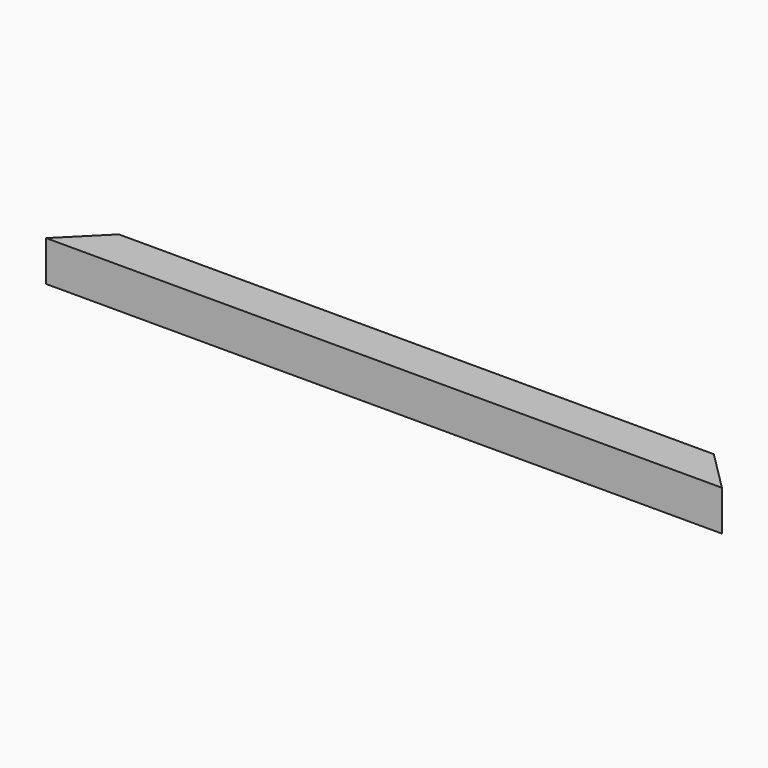
from build123d import *

# Parameters (mm, degrees)
F1_DEPTH = 212.5
F3_DEPTH = 25.4


# Not quite as in the source:
# - a pattern or mirror of a feature is missing from the dataset's text; its kind, count and spacing are read off the source's solid


with BuildPart() as f1:
    # F0 (on Right) → F1 (new body, symmetric)
    with BuildSketch(Plane.YZ):
        Polygon((0, 15.2755248485), (0, -10.1244751515), (3.2, -10.1244751515), (3.2, 12.0755248485), (25.4, 12.0755248485), (25.4, 15.2755248485), align=None)
    extrude(amount=F1_DEPTH, both=True)

    # F2 (on face) → F3 (cut)
    with BuildSketch(Plane.XY.offset(15.2755248485)):
        Polygon((-212.5, 25.4), (-212.5, 0), (-187.1, 25.4), align=None)
    f3 = extrude(amount=-F3_DEPTH, mode=Mode.SUBTRACT)

    # F3_copies: F3 across plane
    add(f3.mirror(Plane(origin=(0, 0, 0), x_dir=(0, 0, 1), z_dir=(1, 0, 0))), mode=Mode.SUBTRACT)


solid = f1.part
